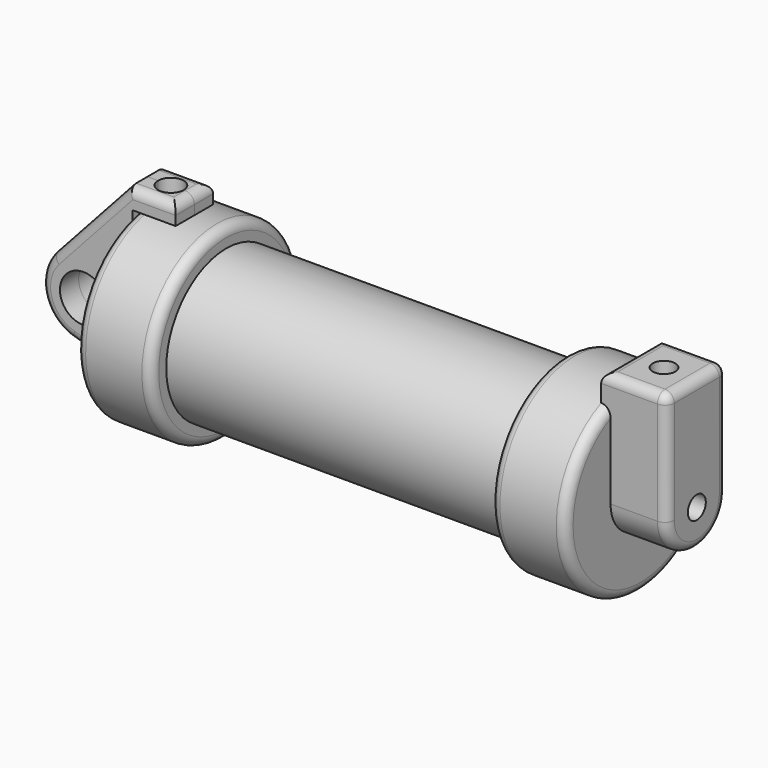
from build123d import *

# Parameters (mm, degrees)
F0_W      = 5.842
F0_H      = 12.7
F0_R      = 3.175
F3_DEPTH  = 3.175
F4_DEPTH  = 3.175
F5_R      = 1.524
F6_DEPTH  = 7.62
F7_DEPTH  = 1.27
F8_DEPTH  = 56.134
F9_R      = 1.524
F10_DEPTH = 10.414
F12_DEPTH = 17.78
F13_DEPTH = 17.78
F14_R     = 1.27
F15_R     = 1.27
F15_2_R   = 1.27
F15_3_R   = 1.27


with BuildPart() as f1:
    # F0 (on Front) → F1 (revolve)
    with BuildSketch(Plane.XZ):
        with Locations((2.921, 6.35)):
            Rectangle(F0_W, F0_H)
    revolve(axis=Axis((33.147, 0, 0), (-1, 0, 0)))

    # F0 (on Front) → F2 (revolve)
    with BuildSketch(Plane.XZ):
        Polygon((5.842, 12.7), (5.842, 0), (66.294, 0), (66.294, 12.7), (56.134, 12.7), (56.134, 10.16), (10.16, 10.16), (10.16, 12.7), align=None)
    revolve(axis=Axis((33.147, 0, 0), (-1, 0, 0)))

    # F5 (on face) → F6 (join)
    with BuildSketch(Plane.YZ.offset(66.294)):
        with BuildLine():
            ThreePointArc((-5.08, 0), (0, -5.08), (5.08, 0))
            ThreePointArc((5.08, 0), (0, 5.08), (-5.08, 0))
        make_face()
        Circle(F5_R, mode=Mode.SUBTRACT)
        with BuildLine():
            ThreePointArc((-5.08, 0), (0, 5.08), (5.08, 0))
            Line((5.08, 0), (5.08, 15.24))
            Line((5.08, 15.24), (-3.2021121588, 15.24))
            Line((-3.2021121588, 15.24), (-5.08, 15.24))
            Line((-5.08, 15.24), (-5.08, 0))
        make_face()
    extrude(amount=F6_DEPTH)

    # F5 (on face) → F7 (join)
    with BuildSketch(Plane.YZ.offset(66.294)):
        with BuildLine():
            ThreePointArc((-5.08, 0), (0, -5.08), (5.08, 0))
            ThreePointArc((5.08, 0), (0, 5.08), (-5.08, 0))
        make_face()
        Circle(F5_R, mode=Mode.SUBTRACT)
        with BuildLine():
            ThreePointArc((-5.08, 0), (0, 5.08), (5.08, 0))
            Line((5.08, 0), (5.08, 15.24))
            Line((5.08, 15.24), (-3.2021121588, 15.24))
            Line((-3.2021121588, 15.24), (-5.08, 15.24))
            Line((-5.08, 15.24), (-5.08, 0))
        make_face()
        Circle(F5_R)
    extrude(amount=-F7_DEPTH)

    # F8 (cut, through all): a face of the model
    f8_faces = [f1.faces().sort_by_distance(p)[0] for p in [
        (66.294, 0, 0),
    ]]
    extrude(f8_faces, amount=-F8_DEPTH, mode=Mode.SUBTRACT)

    # F9 (on face) → F10 (cut)
    with BuildSketch(Plane.XY.offset(15.24)):
        with Locations((69.469, 0)):
            Circle(F9_R)
    extrude(amount=-F10_DEPTH, mode=Mode.SUBTRACT)

    # F14
    f14_edges = [f1.edges().sort_by_distance(p)[0] for p in [
        (10.16, 0, -12.7),
    ]]
    fillet(f14_edges, radius=F14_R)

    # F15
    f15_edges = [f1.edges().sort_by_distance(p)[0] for p in [
        (66.294, 0, -12.7),
        (73.914, 0, 15.24),
        (56.134, 0, -12.7),
        (0, 0, -12.7),
        (69.469, -5.08, 15.24),
        (65.024, 0, 15.24),
        (69.469, 5.08, 15.24),
        (73.914, -5.08, 7.62),
    ]]
    fillet(f15_edges, radius=F15_R)


with BuildPart() as f3:
    # F0 (on Front) → F3 (new body)
    with BuildSketch(Plane.XZ):
        with BuildLine():
            ThreePointArc((-8.1826630726, -5.5069827884), (-3.1957909266, -4.5493385486), (-0.9398, 0))
            ThreePointArc((-0.9398, 0), (-4.5919612295, 5.3297205562), (-10.8806298187, 3.8475430269))
            ThreePointArc((-10.8806298187, 3.8475430269), (-12.1459778134, -1.5837270034), (-8.1826630726, -5.5069827884))
        make_face()
        with Locations((-6.6548, 0)):
            Circle(F0_R, mode=Mode.SUBTRACT)
        with BuildLine():
            Line((5.842, 0), (0, 0))
            Line((0, 0), (-0.9398, 0))
            ThreePointArc((-0.9398, 0), (-3.1957909266, -4.5493385486), (-8.1826630726, -5.5069827884))
            Line((-8.1826630726, -5.5069827884), (5.842, -9.398))
            Line((5.842, -9.398), (5.842, 0))
        make_face()
        with BuildLine():
            Line((-0.9398, 0), (0, 0))
            Line((0, 0), (0, 12.7))
            Line((0, 12.7), (5.842, 12.7))
            Line((5.842, 12.7), (5.842, 15.24))
            Line((5.842, 15.24), (-0.508, 15.24))
            Line((-0.508, 15.24), (-10.8806298187, 3.8475430269))
            ThreePointArc((-10.8806298187, 3.8475430269), (-4.5919612295, 5.3297205562), (-0.9398, 0))
        make_face()
    extrude(amount=F3_DEPTH)

    # F11 (on face) → F13 (cut)
    with BuildSketch(Plane.XY.offset(15.24)):
        with BuildLine():
            ThreePointArc((0.9335704477, 0), (2.667, -1.7334295523), (4.4004295523, 0))
            Line((4.4004295523, 0), (0.9335704477, 0))
        make_face()
    extrude(amount=-F13_DEPTH, mode=Mode.SUBTRACT)

    # F15#2
    f15_2_edges = [f3.edges().sort_by_distance(p)[0] for p in [
        (2.667, -3.175, 15.24),
        (5.842, -1.5875, 15.24),
        (-12.145978, -3.175, -1.583727),
    ]]
    fillet(f15_2_edges, radius=F15_2_R)


with BuildPart() as f4:
    # F0 (on Front) → F4 (new body)
    with BuildSketch(Plane.XZ):
        with BuildLine():
            Line((-0.9398, 0), (0, 0))
            Line((0, 0), (0, 12.7))
            Line((0, 12.7), (5.842, 12.7))
            Line((5.842, 12.7), (5.842, 15.24))
            Line((5.842, 15.24), (-0.508, 15.24))
            Line((-0.508, 15.24), (-10.8806298187, 3.8475430269))
            ThreePointArc((-10.8806298187, 3.8475430269), (-4.5919612295, 5.3297205562), (-0.9398, 0))
        make_face()
        with BuildLine():
            ThreePointArc((-8.1826630726, -5.5069827884), (-3.1957909266, -4.5493385486), (-0.9398, 0))
            ThreePointArc((-0.9398, 0), (-4.5919612295, 5.3297205562), (-10.8806298187, 3.8475430269))
            ThreePointArc((-10.8806298187, 3.8475430269), (-12.1459778134, -1.5837270034), (-8.1826630726, -5.5069827884))
        make_face()
        with Locations((-6.6548, 0)):
            Circle(F0_R, mode=Mode.SUBTRACT)
        with BuildLine():
            Line((5.842, 0), (0, 0))
            Line((0, 0), (-0.9398, 0))
            ThreePointArc((-0.9398, 0), (-3.1957909266, -4.5493385486), (-8.1826630726, -5.5069827884))
            Line((-8.1826630726, -5.5069827884), (5.842, -9.398))
            Line((5.842, -9.398), (5.842, 0))
        make_face()
    extrude(amount=-F4_DEPTH)

    # F11 (on face) → F12 (cut)
    with BuildSketch(Plane.XY.offset(15.24)):
        with BuildLine():
            Line((0.9335704477, 0), (4.4004295523, 0))
            ThreePointArc((4.4004295523, 0), (2.667, 1.7334295523), (0.9335704477, 0))
        make_face()
        with BuildLine():
            ThreePointArc((0.9335704477, 0), (2.667, -1.7334295523), (4.4004295523, 0))
            Line((4.4004295523, 0), (0.9335704477, 0))
        make_face()
    extrude(amount=-F12_DEPTH, mode=Mode.SUBTRACT)

    # F15#3
    f15_3_edges = [f4.edges().sort_by_distance(p)[0] for p in [
        (2.667, 3.175, 15.24),
        (5.842, 1.5875, 15.24),
        (-5.694315, 3.175, 9.543772),
    ]]
    fillet(f15_3_edges, radius=F15_3_R)


solid = Compound([f1.part, f3.part, f4.part])
